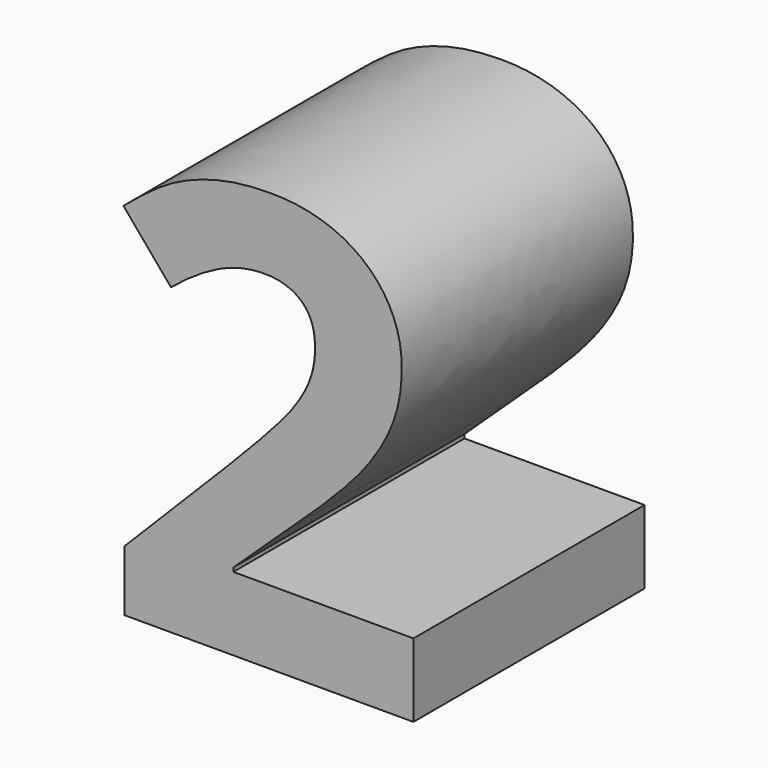
from build123d import *

# Parameters (mm, degrees)
F0_TEXT_SIZE = 50.0869565217
F1_DEPTH     = 25


# Not quite as in the source:
# - Text() gives the source's letters only with a copy of the font that has no kerning and outlines rounded to 1/6400 em; it was checked with that copy


with BuildPart() as f1:
    # F0 (on Front) → F1 (new body)
    with BuildSketch(Plane.XZ):
        with Locations((-10.9794132073, -23.638535158)):
            Text('2', F0_TEXT_SIZE, font='Open Sans', font_style=FontStyle.BOLD, text_align=(TextAlign.LEFT, TextAlign.BOTTOM))
    extrude(amount=F1_DEPTH)


solid = f1.part
